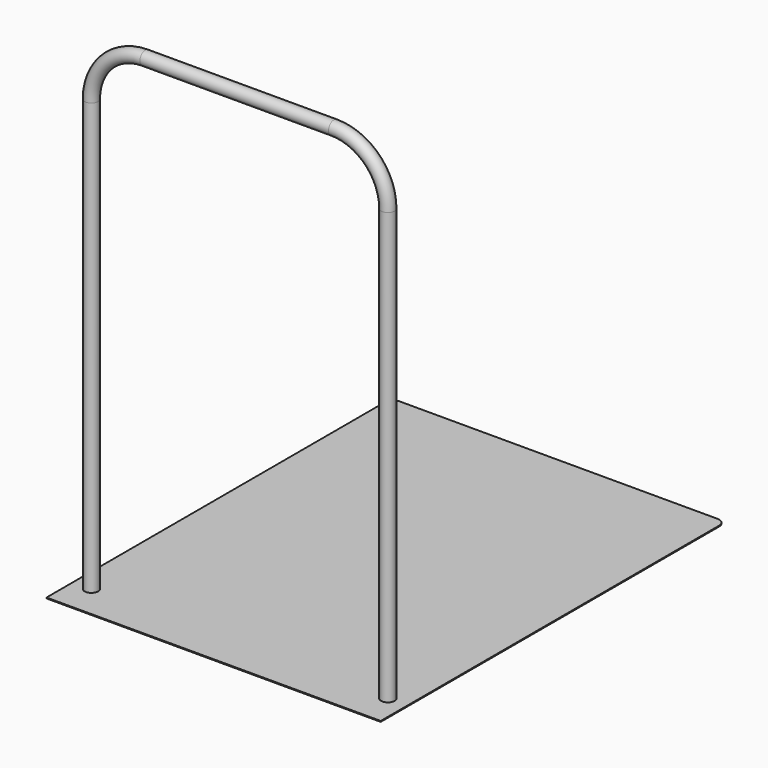
from build123d import *

# Parameters (mm, degrees)
F0_R         = 12.5
F0_R_2       = 10.9
F3_W         = 620
F3_H         = 800
F4_DEPTH     = 1.6
F5_R         = 15
F6_R         = 15
F7_W         = 558.6059093475
F7_H         = 742.6531389356
F8_DEPTH     = 15
F9_W         = 530.512617901
F9_H         = 715.3386492282
F10_DEPTH    = 15
F11_R        = 5
F12_T1_DEPTH = 10
F12_S5_W     = 5.1
F12_S5_H     = 5.1
F12_T6_DEPTH = 5.1


# Not quite as in the source:
# - a fillet or chamfer that OpenCascade refuses, or shapes differently, is made with other operations: its cross-section is extruded or revolved along the edge and cut away or added


with BuildPart() as f2:
    # F2: sweep along a path in F1
    with BuildLine(Plane.XZ) as f2_path:
        Line((0, 0), (0, 800))
        ThreePointArc((0, 800), (29.2893218813, 870.7106781187), (100, 900))
        Line((100, 900), (450, 900))
        ThreePointArc((450, 900), (520.7106781187, 870.7106781187), (550, 800))
        Line((550, 800), (550, 0))
    # F0 (on Top) → F2 (sweep)
    with BuildSketch(Plane.XY):
        Circle(F0_R)
        Circle(F0_R_2, mode=Mode.SUBTRACT)
    sweep(path=f2_path.line)

    # F3 (on Top) → F4 (join)
    with BuildSketch(Plane.XY):
        with Locations((276.0508990288, 338.4082295001)):
            Rectangle(F3_W, F3_H)
    extrude(amount=-F4_DEPTH)

    # F5
    f5_edges = [f2.edges().sort_by_distance(p)[0] for p in [
        (-33.949101, 738.40823, -0.8),
    ]]
    fillet(f5_edges, radius=F5_R)

    # F6
    f6_edges = [f2.edges().sort_by_distance(p)[0] for p in [
        (586.050899, 738.40823, -0.8),
    ]]
    fillet(f6_edges, radius=F6_R)

    # F7 (on face) → F8 (join)
    with BuildSketch(Plane(origin=(0, 0, -1.6), x_dir=(1, 0, 0), z_dir=(0, 0, -1))):
        with Locations((279.3029546738, -329.9668394029)):
            Rectangle(F7_W, F7_H)
    extrude(amount=F8_DEPTH)

    # F9 (on face) → F10 (cut)
    with BuildSketch(Plane(origin=(0, 0, -16.6), x_dir=(1, 0, 0), z_dir=(0, 0, -1))):
        with Locations((281.7520266399, -330.8358481154)):
            Rectangle(F9_W, F9_H)
    extrude(amount=-F10_DEPTH, mode=Mode.SUBTRACT)

    # F11
    f11_edges = [f2.edges().sort_by_distance(p)[0] for p in [
        (558.605909, 329.966839, -16.6),
        (547.008336, 330.835848, -16.6),
        (279.302955, -41.35973, -16.6),
        (281.752027, -26.833476, -16.6),
        (16.495718, 330.835848, -16.6),
        (0, 329.966839, -16.6),
        (281.752027, 688.505173, -16.6),
        (279.302955, 701.293409, -16.6),
        (558.605909, 701.293409, -9.1),
        (0, 701.293409, -9.1),
        (0, -41.35973, -9.1),
    ]]
    fillet(f11_edges, radius=F11_R)

    # F12: fillet of radius 5 on 2 edges, made by hand

    # F12_s2 → F12_t1 (cut)
    with BuildSketch(Plane.XY.offset(-11.6)):
        with BuildLine():
            ThreePointArc((558.6059093475, -36.3597300649), (557.1414432535, -39.8952639708), (553.6059093475, -41.3597300649))
            Line((553.6059093475, -41.3597300649), (558.6059093475, -41.3597300649))
            Line((558.6059093475, -41.3597300649), (558.6059093475, -36.3597300649))
        make_face()
    extrude(amount=F12_T1_DEPTH, mode=Mode.SUBTRACT)


with BuildPart() as f12_tool4:
    # F12_s5 → F12_t6 (new body)
    with BuildSketch(Plane.YZ.offset(553.6059093475)):
        with Locations((-38.9097300649, -14.15)):
            Rectangle(F12_S5_W, F12_S5_H)
    extrude(amount=F12_T6_DEPTH)

    # F12_s7 → F12_t8 (revolve, cut)
    with BuildSketch(Plane(origin=(553.6059093475, -36.3597300649, -11.6), x_dir=(0, 0.7071067812, 0.7071067812), z_dir=(0, 0.7071067812, -0.7071067812))):
        with BuildLine():
            ThreePointArc((0, -5), (5, 0), (0, 5))
            Line((0, 5), (0, -5))
        make_face()
    revolve(axis=Axis((553.6059093475, -36.3597300649, -11.6), (1, 0, 0)), mode=Mode.SUBTRACT)


with BuildPart() as f2_1:
    add(f2.part)

    # F12_t3: cut F12_tool4
    add(f12_tool4.part, mode=Mode.SUBTRACT)


solid = f2_1.part
